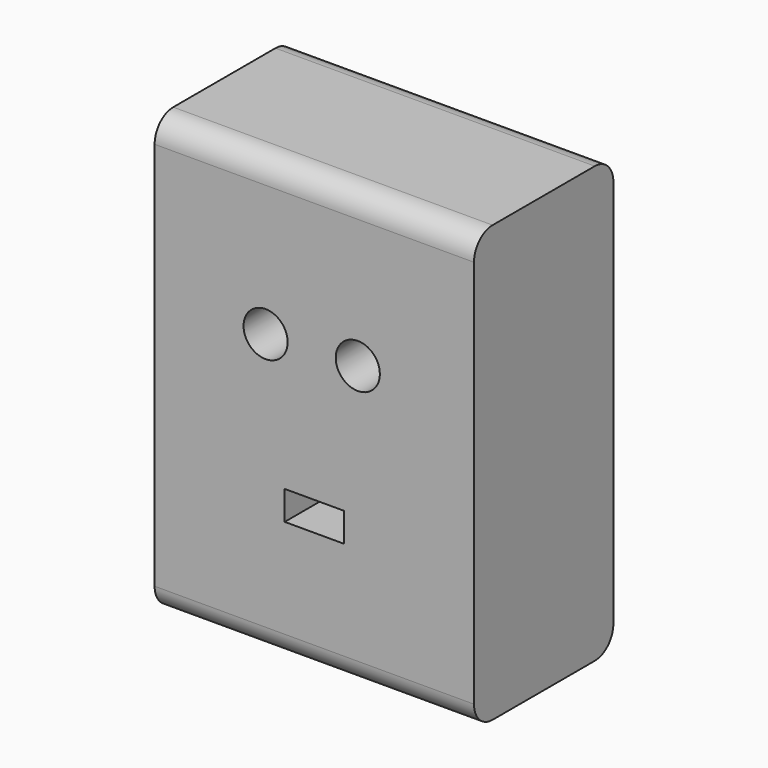
from build123d import *

# Parameters (mm, degrees)
F0_W     = 69.85
F0_H     = 95.25
F1_DEPTH = 38.1
F2_W     = 44.45
F2_H     = 73.66
F3_DEPTH = 25.4
F4_R     = 5.08
F5_R     = 4.826
F6_DEPTH = 12.7
F7_W     = 12.954
F7_H     = 6.35
F8_DEPTH = 12.7


# Not quite as in the source:
# - a feature names something its author has since deleted; it is built from what else it names


with BuildPart() as f1:
    # F0 (on Front) → F1 (new body)
    with BuildSketch(Plane.XZ):
        Rectangle(F0_W, F0_H)
    extrude(amount=F1_DEPTH)

    # F2 (on face) → F3 (cut)
    with BuildSketch(Plane(origin=(0, 0, 0), x_dir=(-1, 0, 0), z_dir=(0, 1, 0))):
        Rectangle(F2_W, F2_H)
    extrude(amount=-F3_DEPTH, mode=Mode.SUBTRACT)

    # F4
    f4_edges = [f1.edges().sort_by_distance(p)[0] for p in [
        (0, -38.1, 47.625),
        (0, 0, 47.625),
        (0, -38.1, -47.625),
        (0, 0, -47.625),
    ]]
    fillet(f4_edges, radius=F4_R)

    # F5 (on face) → F6 (cut)
    with BuildSketch(Plane.XZ.offset(38.1)):
        with Locations((-10.6567444081, 13.887990205)):
            Circle(F5_R)
        with Locations((9.5055226038, 14.3169752002)):
            Circle(F5_R)
    extrude(amount=-F6_DEPTH, mode=Mode.SUBTRACT)

    # F7 (on face) → F8 (cut)
    with BuildSketch(Plane.XZ.offset(38.1)):
        with Locations((0, -17.7338177471)):
            Rectangle(F7_W, F7_H)
    extrude(amount=-F8_DEPTH, mode=Mode.SUBTRACT)


solid = f1.part
